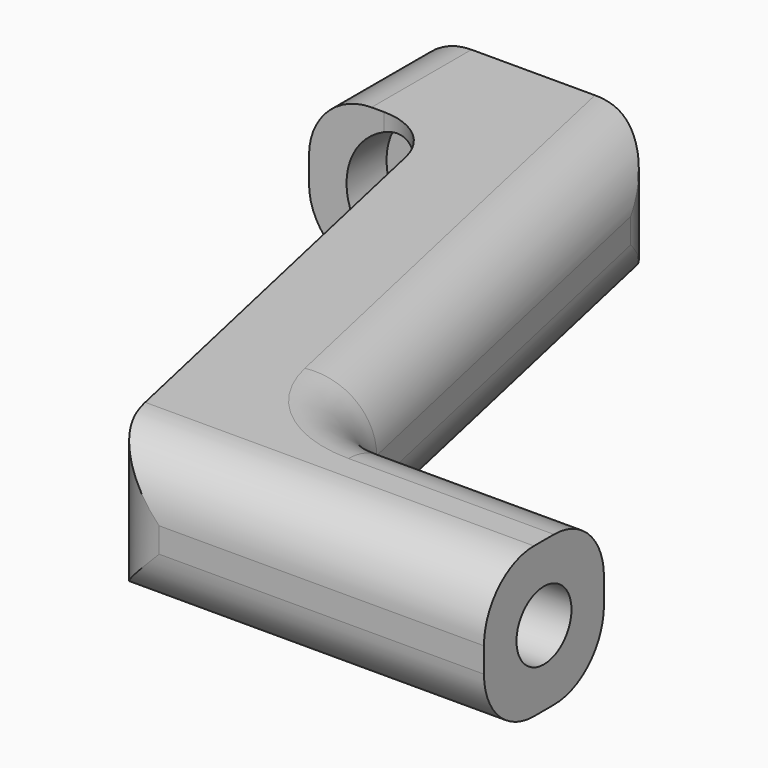
from build123d import *

# Parameters (mm, degrees)
F1_DEPTH     = 12
F3_START     = -10
F2_R         = 2.75
F3_DEPTH     = 40.001
F4_DEPTH     = 50.001
F5_R         = 2.75
F6_DEPTH     = 55.001
F7_START     = -6
F5_R_2       = 5
F7_DEPTH     = 49.001
F8_T1_DEPTH  = 12
F8_T6_DEPTH  = 11.4445693846
F8_S7_R      = 5
F8_T8_DEPTH  = 8
F8_T12_DEPTH = 11.4445693846
F8_S13_R     = 5
F8_T14_DEPTH = 8
F8_T15_DEPTH = 55
F8_T17_DEPTH = 35
F8_T19_DEPTH = 28.9335864126
F8_T21_DEPTH = 32.0542901591
F8_T23_DEPTH = 52.5380765975
F8_T26_ANGLE = 77.4711922908
F8_T28_ANGLE = 77.4711922908


# Not quite as in the source:
# - a fillet or chamfer that OpenCascade refuses, or shapes differently, is made with other operations: its cross-section is extruded or revolved along the edge and cut away or added


with BuildPart() as f1:
    # F0 (on Top) → F1 (new body)
    with BuildSketch(Plane.XY):
        Polygon((-5.2704296331, 25.1133128916), (-25.2704296331, 25.1133128916), (-25.2704296331, 15.1133128916), (-15.2704296331, 15.1133128916), (-5.2704296331, -29.8866871084), (24.7295703669, -29.8866871084), (24.7295703669, -17.8866871084), (4.2851259224, -17.8866871084), align=None)
    extrude(amount=F1_DEPTH)

    # F2 (on face) → F3 (cut)
    with BuildSketch(Plane.YZ.offset(24.7295703669).offset(F3_START)):
        Polygon((-19.6366871084, 3.5462613559), (-19.6366871084, 8.4537386441), (-23.8866871084, 10.9074772881), (-28.1366871084, 8.4537386441), (-28.1366871084, 3.5462613559), (-23.8866871084, 1.0925227119), align=None)
        with Locations((-23.8866871084, 6)):
            Circle(F2_R, mode=Mode.SUBTRACT)
    extrude(amount=-F3_DEPTH, mode=Mode.SUBTRACT)

    # F2 (on face) → F4 (cut, through all)
    with BuildSketch(Plane.YZ.offset(24.7295703669)):
        with Locations((-23.8866871084, 6)):
            Circle(F2_R)
    extrude(amount=-F4_DEPTH, mode=Mode.SUBTRACT)

    # F5 (on face) → F6 (cut, through all)
    with BuildSketch(Plane(origin=(0, 25.1133128916, 0), x_dir=(-1, 0, 0), z_dir=(0, 1, 0))):
        with Locations((17.2704296331, 6)):
            Circle(F5_R)
    extrude(amount=-F6_DEPTH, mode=Mode.SUBTRACT)

    # F5 (on face) → F7 (cut)
    with BuildSketch(Plane(origin=(0, 25.1133128916, 0), x_dir=(-1, 0, 0), z_dir=(0, 1, 0)).offset(F7_START)):
        with Locations((17.2704296331, 6)):
            Circle(F5_R_2)
        with Locations((17.2704296331, 6)):
            Circle(F5_R, mode=Mode.SUBTRACT)
    extrude(amount=-F7_DEPTH, mode=Mode.SUBTRACT)

    # F8: fillet of radius 5 on 13 edges, made by hand

    # F8_s2 → F8_t1 (join)
    with BuildSketch(Plane.XY):
        with BuildLine():
            ThreePointArc((3.4150486533, -13.9713393975), (5.1673469863, -16.7868961698), (8.2959839543, -17.8866871084))
            Line((8.2959839543, -17.8866871084), (4.2851259224, -17.8866871084))
            Line((4.2851259224, -17.8866871084), (3.4150486533, -13.9713393975))
        make_face()
    extrude(amount=F8_T1_DEPTH)


with BuildPart() as f8_tool4:
    # F8_s5 → F8_t6 (new body)
    with BuildSketch(Plane.XY):
        with BuildLine():
            ThreePointArc((-19.281287665, 15.1133128916), (-16.152650697, 14.013521953), (-14.400352364, 11.1979651807))
            Line((-14.400352364, 11.1979651807), (-15.2704296331, 15.1133128916))
            Line((-15.2704296331, 15.1133128916), (-19.281287665, 15.1133128916))
        make_face()
    extrude(amount=F8_T6_DEPTH)

    # F8_s7 → F8_t8 (cut, symmetric)
    with BuildSketch(Plane.XZ.offset(-13.2)):
        with Locations((-17.2704296331, 6)):
            Circle(F8_S7_R)
    extrude(amount=F8_T8_DEPTH, both=True, mode=Mode.SUBTRACT)


with BuildPart() as f1_1:
    add(f1.part)

    # F8_t3: union F8_tool4
    add(f8_tool4.part)


with BuildPart() as f8_tool10:
    # F8_s11 → F8_t12 (new body)
    with BuildSketch(Plane.XY.offset(0.5554306154)):
        with BuildLine():
            ThreePointArc((-19.281287665, 15.1133128916), (-16.152650697, 14.013521953), (-14.400352364, 11.1979651807))
            Line((-14.400352364, 11.1979651807), (-15.2704296331, 15.1133128916))
            Line((-15.2704296331, 15.1133128916), (-19.281287665, 15.1133128916))
        make_face()
    extrude(amount=F8_T12_DEPTH)

    # F8_s13 → F8_t14 (cut, symmetric)
    with BuildSketch(Plane.XZ.offset(-13.2)):
        with Locations((-17.2704296331, 6)):
            Circle(F8_S13_R)
    extrude(amount=F8_T14_DEPTH, both=True, mode=Mode.SUBTRACT)


with BuildPart() as f1_2:
    add(f1_1.part)

    # F8_t9: union F8_tool10
    add(f8_tool10.part)

    # F8_s16 → F8_t15 (cut)
    with BuildSketch(Plane.YZ.offset(-17.7704296331)):
        with BuildLine():
            ThreePointArc((-29.8866871084, 7), (-28.4222210144, 10.5355339059), (-24.8866871084, 12))
            Line((-24.8866871084, 12), (-29.8866871084, 12))
            Line((-29.8866871084, 12), (-29.8866871084, 7))
        make_face()
        with BuildLine():
            ThreePointArc((-29.8866871084, 5), (-28.4222210144, 1.4644660941), (-24.8866871084, 0))
            Line((-24.8866871084, 0), (-29.8866871084, 0))
            Line((-29.8866871084, 0), (-29.8866871084, 5))
        make_face()
    extrude(amount=F8_T15_DEPTH, mode=Mode.SUBTRACT)

    # F8_s18 → F8_t17 (cut)
    with BuildSketch(Plane.XZ.offset(-37.6133128916)):
        with BuildLine():
            ThreePointArc((-25.2704296331, 7), (-23.8059635391, 10.5355339059), (-20.2704296331, 12))
            Line((-20.2704296331, 12), (-25.2704296331, 12))
            Line((-25.2704296331, 12), (-25.2704296331, 7))
        make_face()
        with BuildLine():
            ThreePointArc((-25.2704296331, 5), (-23.8059635391, 1.4644660941), (-20.2704296331, 0))
            Line((-20.2704296331, 0), (-25.2704296331, 0))
            Line((-25.2704296331, 0), (-25.2704296331, 5))
        make_face()
    extrude(amount=F8_T17_DEPTH, mode=Mode.SUBTRACT)

    # F8_s20 → F8_t19 (cut)
    with BuildSketch(Plane.YZ.offset(8.2959839543)):
        with BuildLine():
            ThreePointArc((-17.8866871084, 7), (-19.3511532025, 10.5355339059), (-22.8866871084, 12))
            Line((-22.8866871084, 12), (-17.8866871084, 12))
            Line((-17.8866871084, 12), (-17.8866871084, 7))
        make_face()
        with BuildLine():
            ThreePointArc((-17.8866871084, 5), (-19.3511532025, 1.4644660941), (-22.8866871084, 0))
            Line((-22.8866871084, 0), (-17.8866871084, 0))
            Line((-17.8866871084, 0), (-17.8866871084, 5))
        make_face()
    extrude(amount=F8_T19_DEPTH, mode=Mode.SUBTRACT)

    # F8_s22 → F8_t21 (cut)
    with BuildSketch(Plane.XY.offset(-10.0271450796)):
        with BuildLine():
            ThreePointArc((-6.1405069022, -25.9713393975), (-4.3882085693, -28.7868961698), (-1.2595716013, -29.8866871084))
            Line((-1.2595716013, -29.8866871084), (-5.2704296331, -29.8866871084))
            Line((-5.2704296331, -29.8866871084), (-6.1405069022, -25.9713393975))
        make_face()
        with BuildLine():
            ThreePointArc((-9.281287665, 25.1133128916), (-6.152650697, 24.013521953), (-4.400352364, 21.1979651807))
            Line((-4.400352364, 21.1979651807), (-5.2704296331, 25.1133128916))
            Line((-5.2704296331, 25.1133128916), (-9.281287665, 25.1133128916))
        make_face()
    extrude(amount=F8_T21_DEPTH, mode=Mode.SUBTRACT)

    # F8_s24 → F8_t23 (cut)
    with BuildSketch(Plane(origin=(3.1193447502, -14.037051376, 0), x_dir=(0, 0, 1), z_dir=(-0.2169304578, 0.9761870602, 0))):
        with BuildLine():
            ThreePointArc((0, -4.6970827466), (1.4644660941, -1.1615488406), (5, 0.3029172534))
            Line((5, 0.3029172534), (0, 0.3029172534))
            Line((0, 0.3029172534), (0, -4.6970827466))
        make_face()
        with BuildLine():
            ThreePointArc((12, -4.6970827466), (10.5355339059, -1.1615488406), (7, 0.3029172534))
            Line((7, 0.3029172534), (12, 0.3029172534))
            Line((12, 0.3029172534), (12, -4.6970827466))
        make_face()
    extrude(amount=F8_T23_DEPTH, mode=Mode.SUBTRACT)

    # F8_s25 → F8_t26 (revolve, cut)
    with BuildSketch(Plane(origin=(3.1193447502, -14.037051376, 0), x_dir=(0, 0, 1), z_dir=(-0.2169304578, 0.9761870602, 0))):
        with BuildLine():
            ThreePointArc((7, 0.3029172534), (10.5355339059, -1.1615488406), (12, -4.6970827466))
            Line((12, -4.6970827466), (12, 0.3029172534))
            Line((12, 0.3029172534), (7, 0.3029172534))
        make_face()
    revolve(axis=Axis((8.2959839543, -12.8866871084, 12), (0, 0, 1)), revolution_arc=F8_T26_ANGLE, mode=Mode.SUBTRACT)

    # F8_s27 → F8_t28 (revolve, cut)
    with BuildSketch(Plane(origin=(3.1193447502, -14.037051376, 0), x_dir=(0, 0, 1), z_dir=(-0.2169304578, 0.9761870602, 0))):
        with BuildLine():
            ThreePointArc((5, 0.3029172534), (1.4644660941, -1.1615488406), (0, -4.6970827466))
            Line((0, -4.6970827466), (0, 0.3029172534))
            Line((0, 0.3029172534), (5, 0.3029172534))
        make_face()
    revolve(axis=Axis((8.2959839543, -12.8866871084, 0), (0, 0, 1)), revolution_arc=F8_T28_ANGLE, mode=Mode.SUBTRACT)


solid = f1_2.part
